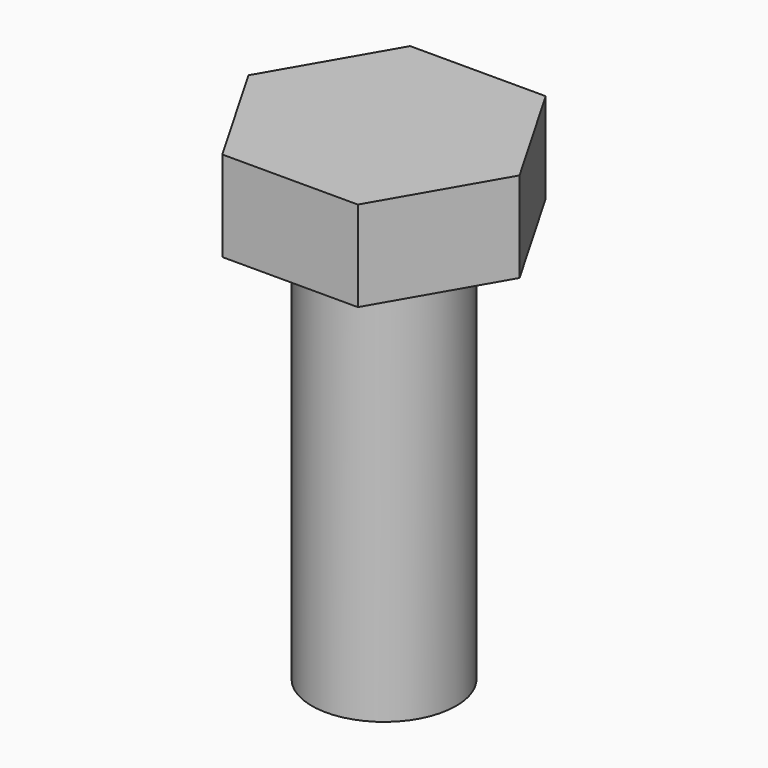
from build123d import *

# Parameters (mm, degrees)
F0_R     = 12.7
F1_DEPTH = 69.85
F3_DEPTH = 15.875


# Not quite as in the source:
# - a feature names something its author has since deleted; it is built from what else it names


with BuildPart() as f1:
    # F0 (on Top) → F1 (new body)
    with BuildSketch(Plane.XY):
        Circle(F0_R)
    extrude(amount=-F1_DEPTH)

    # F2 (on face) → F3 (join)
    with BuildSketch(Plane.XY):
        Polygon((11.9150661804, 20.6375), (-11.9150661804, 20.6375), (-23.8301323608, 0), (-11.9150661804, -20.6375), (11.9150661804, -20.6375), (23.8301323608, 0), align=None)
    extrude(amount=F3_DEPTH)


solid = f1.part
